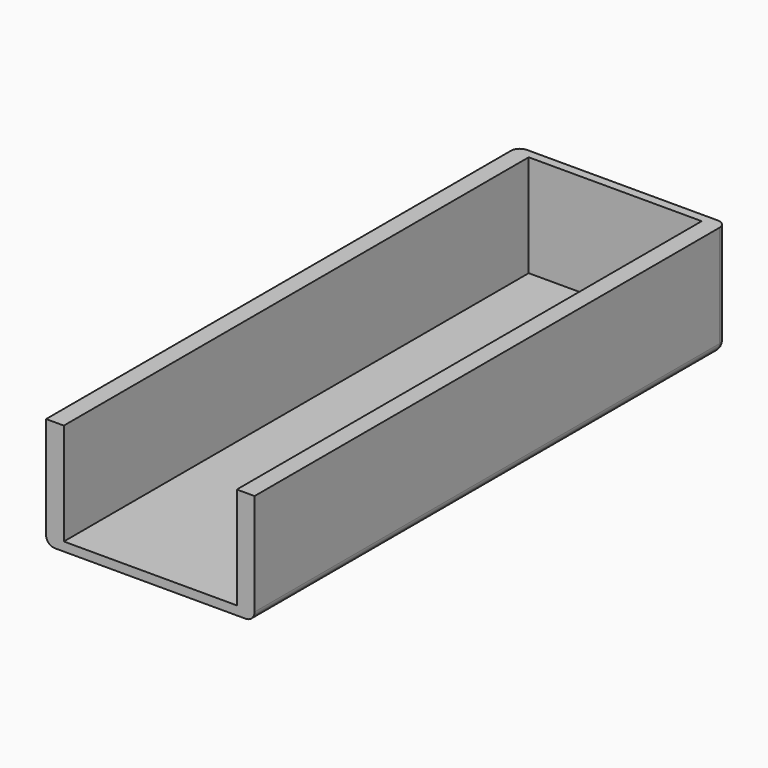
from build123d import *

# Parameters (mm, degrees)
F0_W        = 47
F0_H        = 133
F1_DEPTH    = 25
F2_W        = 41
F2_H        = 23
F3_DEPTH    = 131
F4_R        = 2
F5_R        = 2
F6_T1_DEPTH = 28
F6_S5_W     = 2
F6_S5_H     = 2
F6_T6_DEPTH = 2
F7_DEPTH    = 1
F8_DEPTH    = 1
F9_DEPTH    = 0.5


# Not quite as in the source:
# - a fillet or chamfer that OpenCascade refuses, or shapes differently, is made with other operations: its cross-section is extruded or revolved along the edge and cut away or added


with BuildPart() as f1:
    # F0 (on Top) → F1 (new body)
    with BuildSketch(Plane.XY):
        with Locations((-1.0670694858, 16.9100829363)):
            Rectangle(F0_W, F0_H)
    extrude(amount=F1_DEPTH)

    # F2 (on face) → F3 (cut, through all)
    with BuildSketch(Plane.XZ.offset(49.5899170637)):
        with Locations((-1.0670694858, 13.5)):
            Rectangle(F2_W, F2_H)
    extrude(amount=-F3_DEPTH, mode=Mode.SUBTRACT)

    # F4
    f4_edges = [f1.edges().sort_by_distance(p)[0] for p in [
        (22.432931, 16.910083, 0),
        (-1.067069, 83.410083, 0),
    ]]
    fillet(f4_edges, radius=F4_R)

    # F5
    f5_edges = [f1.edges().sort_by_distance(p)[0] for p in [
        (-24.567069, 15.910083, 0),
    ]]
    fillet(f5_edges, radius=F5_R)

    # F6: fillet of radius 2 on 1 edges, made by hand

    # F6_s2 → F6_t1 (cut)
    with BuildSketch(Plane.XY.offset(2)):
        with BuildLine():
            ThreePointArc((20.4329305142, 83.4100829363), (21.8471440766, 82.8242964987), (22.4329305142, 81.4100829363))
            Line((22.4329305142, 81.4100829363), (22.4329305142, 83.4100829363))
            Line((22.4329305142, 83.4100829363), (20.4329305142, 83.4100829363))
        make_face()
    extrude(amount=F6_T1_DEPTH, mode=Mode.SUBTRACT)


with BuildPart() as f6_tool4:
    # F6_s5 → F6_t6 (new body)
    with BuildSketch(Plane.XZ.offset(-81.4100829363)):
        with Locations((21.4329305142, 1)):
            Rectangle(F6_S5_W, F6_S5_H)
    extrude(amount=-F6_T6_DEPTH)

    # F6_s7 → F6_t8 (revolve, cut)
    with BuildSketch(Plane(origin=(20.4329305142, 81.4100829363, 2), x_dir=(-0.7071067812, 0, 0.7071067812), z_dir=(-0.7071067812, 0, -0.7071067812))):
        with BuildLine():
            ThreePointArc((0, -2), (2, 0), (0, 2))
            Line((0, 2), (0, -2))
        make_face()
    revolve(axis=Axis((20.4329305142, 81.4100829363, 2), (0, 1, 0)), mode=Mode.SUBTRACT)


with BuildPart() as f1_1:
    add(f1.part)

    # F6_t3: cut F6_tool4
    add(f6_tool4.part, mode=Mode.SUBTRACT)

    # F7 (add): a face of the model
    f7_faces = [f1_1.faces().sort_by_distance(p)[0] for p in [
        (-21.5670694858, 15.9100829363, 13.5),
    ]]
    extrude(f7_faces, amount=F7_DEPTH)

    # F8 (add): a face of the model
    f8_faces = [f1_1.faces().sort_by_distance(p)[0] for p in [
        (19.4329305142, 15.9100829363, 13.5),
    ]]
    extrude(f8_faces, amount=F8_DEPTH)

    # F9 (add): a face of the model
    f9_faces = [f1_1.faces().sort_by_distance(p)[0] for p in [
        (-20.5670694858, 15.9100829363, 13.5),
    ]]
    extrude(f9_faces, amount=-F9_DEPTH)


solid = f1_1.part
